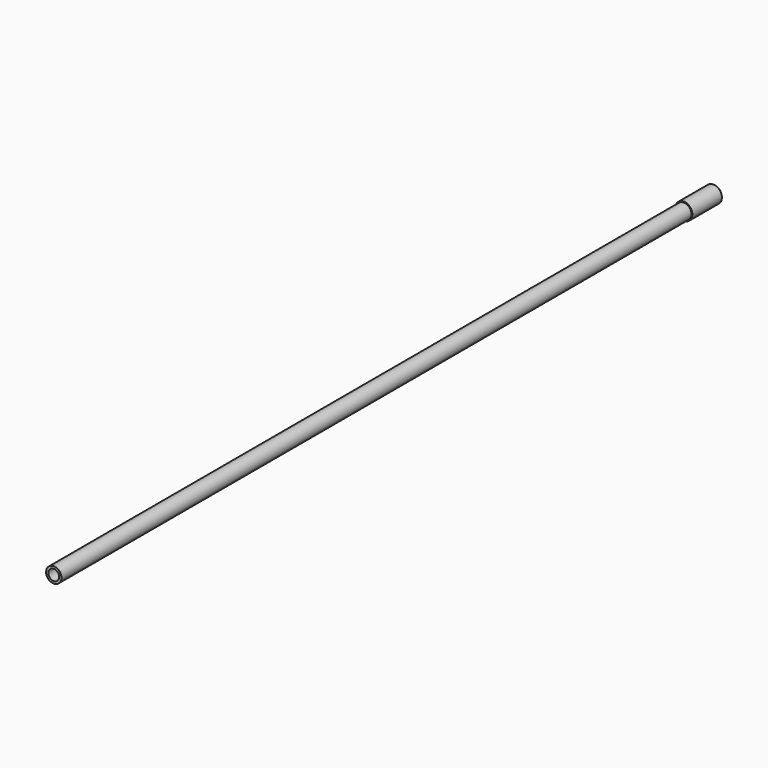
from build123d import *

# Parameters (mm, degrees)
F0_R     = 4.25
F0_R_2   = 3
F1_DEPTH = 456
F2_R     = 4.75
F2_R_2   = 4.25
F2_R_3   = 3.25
F3_DEPTH = 1
F4_DEPTH = 20.5


with BuildPart() as f1:
    # F0 (on Front) → F1 (new body)
    with BuildSketch(Plane.XZ):
        Circle(F0_R)
        Circle(F0_R_2, mode=Mode.SUBTRACT)
    extrude(amount=F1_DEPTH)


with BuildPart() as f3:
    # F2 (on Front) → F3 (new body)
    with BuildSketch(Plane.XZ):
        Circle(F2_R)
        Circle(F2_R_2, mode=Mode.SUBTRACT)
        Circle(F2_R_2)
        Circle(F2_R_3, mode=Mode.SUBTRACT)
    extrude(amount=-F3_DEPTH)

    # F4 (add): a face of the model
    f4_faces = [f3.faces().sort_by_distance(p)[0] for p in [
        (-4.6156497116, 1, 0),
    ]]
    extrude(f4_faces, amount=-F4_DEPTH)

    # F5 (on Right) → F6 (revolve)
    with BuildSketch(Plane.YZ):
        Polygon((1, 3.25), (3, 2.25), (3, 2.75), (1, 3.75), align=None)
    revolve(axis=Axis((0, 3.2308421517, 0), (0, 1, 0)))


solid = Compound([f1.part, f3.part])
